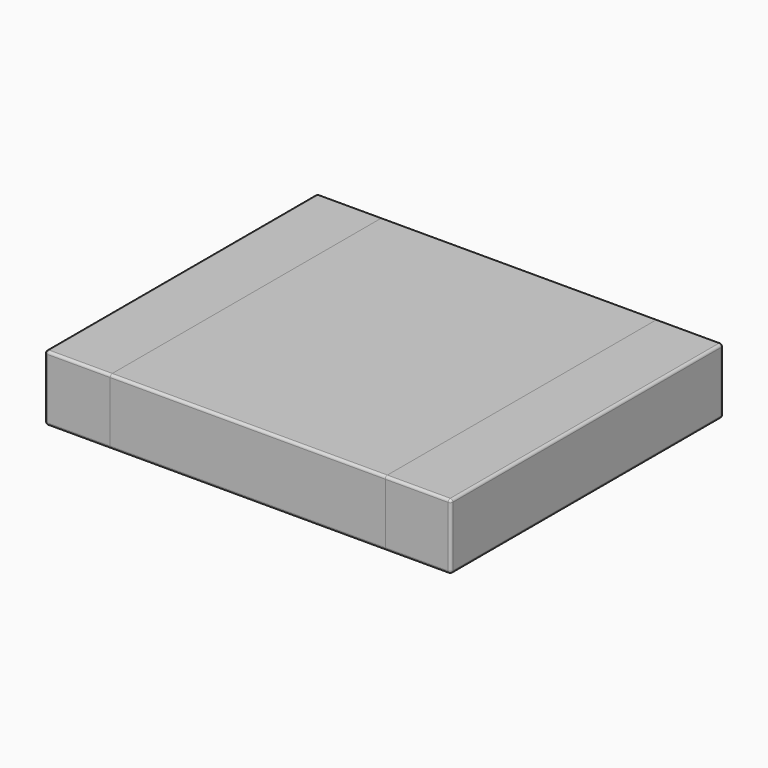
from build123d import *

# Parameters (mm, degrees)
F2_W     = 2.1
F2_H     = 2.6
F3_DEPTH = 0.48
F2_W_2   = 0.5
F4_DEPTH = 0.5
F5_DEPTH = 0.5
F6_DEPTH = 0.02
F7_R     = 0.01999
F7_2_R   = 0.01999
F7_3_R   = 0.01999
F7_4_R   = 0.01999


# Not quite as in the source:
# - a fillet or chamfer is up to 0.001 mm smaller than in the source, because OpenCascade refuses the exact size


with BuildPart() as f3:
    # F2 (on Top) → F3 (new body)
    with BuildSketch(Plane.XY):
        Rectangle(F2_W, F2_H)
    extrude(amount=F3_DEPTH)


with BuildPart() as f4:
    # F2 (on Top) → F4 (new body)
    with BuildSketch(Plane.XY):
        with Locations((-1.3, 0)):
            Rectangle(F2_W_2, F2_H)
    extrude(amount=F4_DEPTH)

    # F7 (radius 0.02 in the source; OpenCascade refuses exactly that, so slightly less here)
    f7_edges = [f4.edges().sort_by_distance(p)[0] for p in [
        (-1.3, -1.3, 0.5),
        (-1.55, 1.3, 0.25),
        (-1.55, -1.3, 0.25),
        (-1.55, 0, 0),
        (-1.55, 0, 0.5),
        (-1.3, 1.3, 0.5),
        (-1.3, 1.3, 0),
        (-1.3, -1.3, 0),
    ]]
    fillet(f7_edges, radius=F7_R)


with BuildPart() as f5:
    # F2 (on Top) → F5 (new body)
    with BuildSketch(Plane.XY):
        with Locations((1.3, 0)):
            Rectangle(F2_W_2, F2_H)
    extrude(amount=F5_DEPTH)

    # F7#2 (radius 0.02 in the source; OpenCascade refuses exactly that, so slightly less here)
    f7_2_edges = [f5.edges().sort_by_distance(p)[0] for p in [
        (1.3, -1.3, 0.5),
        (1.55, -1.3, 0.25),
        (1.55, 1.3, 0.25),
        (1.55, 0, 0),
        (1.55, 0, 0.5),
        (1.3, 1.3, 0.5),
        (1.3, 1.3, 0),
        (1.3, -1.3, 0),
    ]]
    fillet(f7_2_edges, radius=F7_2_R)


with BuildPart() as f6:
    # F6 (new): a face of the model
    f6_faces = [f3.part.faces().sort_by_distance(p)[0] for p in [
        (0, 0, 0.48),
    ]]
    extrude(f6_faces, amount=F6_DEPTH)

    # F7#4 (radius 0.02 in the source; OpenCascade refuses exactly that, so slightly less here)
    f7_4_edges = [f6.edges().sort_by_distance(p)[0] for p in [
        (0, -1.3, 0.5),
        (0, 1.3, 0.5),
    ]]
    fillet(f7_4_edges, radius=F7_4_R)


with BuildPart() as f3_1:
    add(f3.part)

    # F7#3 (radius 0.02 in the source; OpenCascade refuses exactly that, so slightly less here)
    f7_3_edges = [f3_1.edges().sort_by_distance(p)[0] for p in [
        (0, 1.3, 0),
        (0, -1.3, 0),
    ]]
    fillet(f7_3_edges, radius=F7_3_R)


solid = Compound([f4.part, f5.part, f6.part, f3_1.part])
